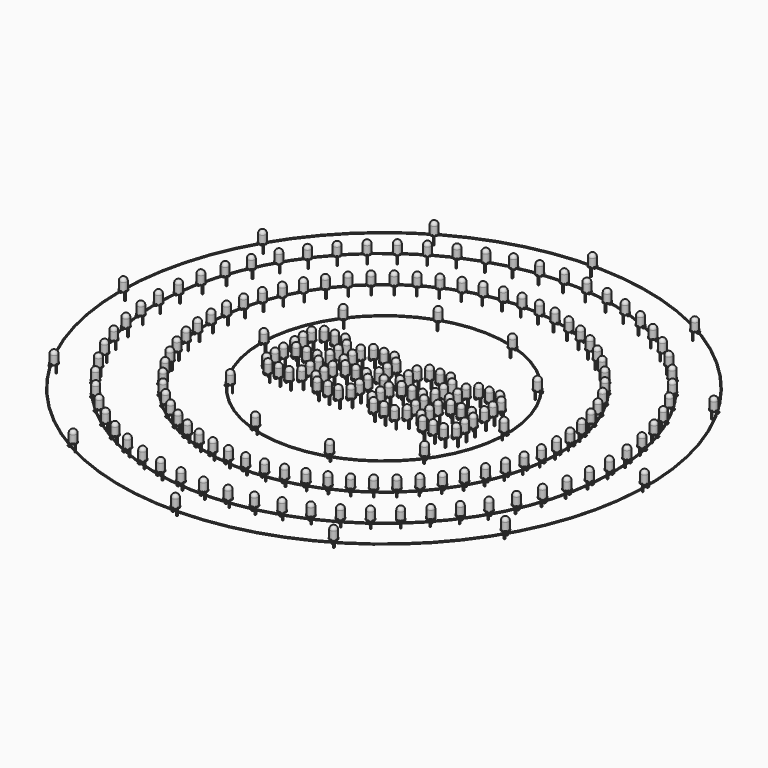
from build123d import *

# Parameters (mm, degrees)
F2_W       = 0.762
F2_H       = 0.762
F3_DEPTH   = 1.27
F4_DEPTH   = 6.35
F5_R       = 0.4064
F7_ANGLE   = 270
F3_FACE1_W = 0.762
F3_FACE1_H = 0.762
F9_ANGLE   = 180
F14_COUNT  = 10
F14_ANGLE  = 324
F15_COUNT  = 60
F15_ANGLE  = 354
F16_COUNT  = 12
F16_ANGLE  = 330


with BuildPart() as f1:
    # F0 (on Top) → F1 (revolve)
    with BuildSketch(Plane.XY):
        with BuildLine():
            Line((-2.794, 0), (0, 0))
            Line((0, 0), (0, 8.636))
            ThreePointArc((0, 8.636), (-1.7960512242, 7.8920512242), (-2.54, 6.096))
            Line((-2.54, 6.096), (-2.54, 0.508))
            Line((-2.54, 0.508), (-2.794, 0.508))
            Line((-2.794, 0.508), (-2.794, 0))
        make_face()
    revolve(axis=Axis((0, 4.318, 0), (0, -1, 0)))

    # F2 (on face) → F3 (join)
    with BuildSketch(Plane.XZ):
        with Locations((-1.27, 0)):
            Rectangle(F2_W, F2_H)
    extrude(amount=F3_DEPTH)

    # F2 (on face) → F4 (join)
    with BuildSketch(Plane.XZ):
        with Locations((1.27, 0)):
            Rectangle(F2_W, F2_H)
    extrude(amount=F4_DEPTH)


with BuildPart() as f6:
    # F5 (on Front) → F6 (revolve)
    with BuildSketch(Plane.XZ):
        with Locations((-190.5, 0)):
            Circle(F5_R)
    revolve(axis=Axis((0, 0, -20.106445998), (0, 0, -1)))


with BuildPart() as f6b:
    # F5 (on Front) → F6, piece 2 (revolve)
    with BuildSketch(Plane.XZ):
        with Locations((-165.1, 0)):
            Circle(F5_R)
    revolve(axis=Axis((0, 0, -20.106445998), (0, 0, -1)))


with BuildPart() as f6c:
    # F5 (on Front) → F6, piece 3 (revolve)
    with BuildSketch(Plane.XZ):
        with Locations((-127, 0)):
            Circle(F5_R)
    revolve(axis=Axis((0, 0, -20.106445998), (0, 0, -1)))


with BuildPart() as f6d:
    # F5 (on Front) → F6, piece 4 (revolve)
    with BuildSketch(Plane.XZ):
        with Locations((-88.9, 0)):
            Circle(F5_R)
    revolve(axis=Axis((0, 0, -20.106445998), (0, 0, -1)))


with BuildPart() as f1_1:
    # F7: moved
    add(f1.part.rotate(Axis((-1.397, 0, 0), (-1, 0, 0)), F7_ANGLE))

    # F3_face1 (on face) → F9 (revolve)
    with BuildSketch(Plane(origin=(-1.27, 0, -1.27), x_dir=(1, 0, 0), z_dir=(0, 0, -1))):
        Rectangle(F3_FACE1_W, F3_FACE1_H)
    revolve(axis=Axis((-2.0574, -0.381, -1.27), (0, 1, 0)), revolution_arc=F9_ANGLE)


with BuildPart() as f10_1:
    # F10: copy of F1
    add(f1_1.part.moved(Location((-86.868, 0, 1.27))))


with BuildPart() as f11_1:
    # F11: copy of F1
    add(f1_1.part.moved(Location((-124.968, 0, 1.27))))


with BuildPart() as f12_1:
    # F12: copy of F1
    add(f1_1.part.moved(Location((-163.068, 0, 1.27))))


with BuildPart() as f13_1:
    # F13: copy of F1
    add(f1_1.part.moved(Location((-188.468, 0, 1.27))))


with BuildPart() as f14_1:
    # F14: instance of F10_1
    add(f10_1.part.rotate(Axis((0, 0, 22.3142132163), (0, 0, -1)), 1 * F14_ANGLE / (F14_COUNT - 1)))


with BuildPart() as f14_2:
    # F14: instance of F10_1
    add(f10_1.part.rotate(Axis((0, 0, 22.3142132163), (0, 0, -1)), 2 * F14_ANGLE / (F14_COUNT - 1)))


with BuildPart() as f14_3:
    # F14: instance of F10_1
    add(f10_1.part.rotate(Axis((0, 0, 22.3142132163), (0, 0, -1)), 3 * F14_ANGLE / (F14_COUNT - 1)))


with BuildPart() as f14_4:
    # F14: instance of F10_1
    add(f10_1.part.rotate(Axis((0, 0, 22.3142132163), (0, 0, -1)), 4 * F14_ANGLE / (F14_COUNT - 1)))


with BuildPart() as f14_5:
    # F14: instance of F10_1
    add(f10_1.part.rotate(Axis((0, 0, 22.3142132163), (0, 0, -1)), 5 * F14_ANGLE / (F14_COUNT - 1)))


with BuildPart() as f14_6:
    # F14: instance of F10_1
    add(f10_1.part.rotate(Axis((0, 0, 22.3142132163), (0, 0, -1)), 6 * F14_ANGLE / (F14_COUNT - 1)))


with BuildPart() as f14_7:
    # F14: instance of F10_1
    add(f10_1.part.rotate(Axis((0, 0, 22.3142132163), (0, 0, -1)), 7 * F14_ANGLE / (F14_COUNT - 1)))


with BuildPart() as f14_8:
    # F14: instance of F10_1
    add(f10_1.part.rotate(Axis((0, 0, 22.3142132163), (0, 0, -1)), 8 * F14_ANGLE / (F14_COUNT - 1)))


with BuildPart() as f14_9:
    # F14: instance of F10_1
    add(f10_1.part.rotate(Axis((0, 0, 22.3142132163), (0, 0, -1)), 9 * F14_ANGLE / (F14_COUNT - 1)))


with BuildPart() as f15_1:
    # F15: instance of F11_1
    add(f11_1.part.rotate(Axis((0, 0, 22.3142132163), (0, 0, -1)), 1 * F15_ANGLE / (F15_COUNT - 1)))


with BuildPart() as f15_2:
    # F15: instance of F11_1
    add(f11_1.part.rotate(Axis((0, 0, 22.3142132163), (0, 0, -1)), 2 * F15_ANGLE / (F15_COUNT - 1)))


with BuildPart() as f15_3:
    # F15: instance of F11_1
    add(f11_1.part.rotate(Axis((0, 0, 22.3142132163), (0, 0, -1)), 3 * F15_ANGLE / (F15_COUNT - 1)))


with BuildPart() as f15_4:
    # F15: instance of F11_1
    add(f11_1.part.rotate(Axis((0, 0, 22.3142132163), (0, 0, -1)), 4 * F15_ANGLE / (F15_COUNT - 1)))


with BuildPart() as f15_5:
    # F15: instance of F11_1
    add(f11_1.part.rotate(Axis((0, 0, 22.3142132163), (0, 0, -1)), 5 * F15_ANGLE / (F15_COUNT - 1)))


with BuildPart() as f15_6:
    # F15: instance of F11_1
    add(f11_1.part.rotate(Axis((0, 0, 22.3142132163), (0, 0, -1)), 6 * F15_ANGLE / (F15_COUNT - 1)))


with BuildPart() as f15_7:
    # F15: instance of F11_1
    add(f11_1.part.rotate(Axis((0, 0, 22.3142132163), (0, 0, -1)), 7 * F15_ANGLE / (F15_COUNT - 1)))


with BuildPart() as f15_8:
    # F15: instance of F11_1
    add(f11_1.part.rotate(Axis((0, 0, 22.3142132163), (0, 0, -1)), 8 * F15_ANGLE / (F15_COUNT - 1)))


with BuildPart() as f15_9:
    # F15: instance of F11_1
    add(f11_1.part.rotate(Axis((0, 0, 22.3142132163), (0, 0, -1)), 9 * F15_ANGLE / (F15_COUNT - 1)))


with BuildPart() as f15_10:
    # F15: instance of F11_1
    add(f11_1.part.rotate(Axis((0, 0, 22.3142132163), (0, 0, -1)), 10 * F15_ANGLE / (F15_COUNT - 1)))


with BuildPart() as f15_11:
    # F15: instance of F11_1
    add(f11_1.part.rotate(Axis((0, 0, 22.3142132163), (0, 0, -1)), 11 * F15_ANGLE / (F15_COUNT - 1)))


with BuildPart() as f15_12:
    # F15: instance of F11_1
    add(f11_1.part.rotate(Axis((0, 0, 22.3142132163), (0, 0, -1)), 12 * F15_ANGLE / (F15_COUNT - 1)))


with BuildPart() as f15_13:
    # F15: instance of F11_1
    add(f11_1.part.rotate(Axis((0, 0, 22.3142132163), (0, 0, -1)), 13 * F15_ANGLE / (F15_COUNT - 1)))


with BuildPart() as f15_14:
    # F15: instance of F11_1
    add(f11_1.part.rotate(Axis((0, 0, 22.3142132163), (0, 0, -1)), 14 * F15_ANGLE / (F15_COUNT - 1)))


with BuildPart() as f15_15:
    # F15: instance of F11_1
    add(f11_1.part.rotate(Axis((0, 0, 22.3142132163), (0, 0, -1)), 15 * F15_ANGLE / (F15_COUNT - 1)))


with BuildPart() as f15_16:
    # F15: instance of F11_1
    add(f11_1.part.rotate(Axis((0, 0, 22.3142132163), (0, 0, -1)), 16 * F15_ANGLE / (F15_COUNT - 1)))


with BuildPart() as f15_17:
    # F15: instance of F11_1
    add(f11_1.part.rotate(Axis((0, 0, 22.3142132163), (0, 0, -1)), 17 * F15_ANGLE / (F15_COUNT - 1)))


with BuildPart() as f15_18:
    # F15: instance of F11_1
    add(f11_1.part.rotate(Axis((0, 0, 22.3142132163), (0, 0, -1)), 18 * F15_ANGLE / (F15_COUNT - 1)))


with BuildPart() as f15_19:
    # F15: instance of F11_1
    add(f11_1.part.rotate(Axis((0, 0, 22.3142132163), (0, 0, -1)), 19 * F15_ANGLE / (F15_COUNT - 1)))


with BuildPart() as f15_20:
    # F15: instance of F11_1
    add(f11_1.part.rotate(Axis((0, 0, 22.3142132163), (0, 0, -1)), 20 * F15_ANGLE / (F15_COUNT - 1)))


with BuildPart() as f15_21:
    # F15: instance of F11_1
    add(f11_1.part.rotate(Axis((0, 0, 22.3142132163), (0, 0, -1)), 21 * F15_ANGLE / (F15_COUNT - 1)))


with BuildPart() as f15_22:
    # F15: instance of F11_1
    add(f11_1.part.rotate(Axis((0, 0, 22.3142132163), (0, 0, -1)), 22 * F15_ANGLE / (F15_COUNT - 1)))


with BuildPart() as f15_23:
    # F15: instance of F11_1
    add(f11_1.part.rotate(Axis((0, 0, 22.3142132163), (0, 0, -1)), 23 * F15_ANGLE / (F15_COUNT - 1)))


with BuildPart() as f15_24:
    # F15: instance of F11_1
    add(f11_1.part.rotate(Axis((0, 0, 22.3142132163), (0, 0, -1)), 24 * F15_ANGLE / (F15_COUNT - 1)))


with BuildPart() as f15_25:
    # F15: instance of F11_1
    add(f11_1.part.rotate(Axis((0, 0, 22.3142132163), (0, 0, -1)), 25 * F15_ANGLE / (F15_COUNT - 1)))


with BuildPart() as f15_26:
    # F15: instance of F11_1
    add(f11_1.part.rotate(Axis((0, 0, 22.3142132163), (0, 0, -1)), 26 * F15_ANGLE / (F15_COUNT - 1)))


with BuildPart() as f15_27:
    # F15: instance of F11_1
    add(f11_1.part.rotate(Axis((0, 0, 22.3142132163), (0, 0, -1)), 27 * F15_ANGLE / (F15_COUNT - 1)))


with BuildPart() as f15_28:
    # F15: instance of F11_1
    add(f11_1.part.rotate(Axis((0, 0, 22.3142132163), (0, 0, -1)), 28 * F15_ANGLE / (F15_COUNT - 1)))


with BuildPart() as f15_29:
    # F15: instance of F11_1
    add(f11_1.part.rotate(Axis((0, 0, 22.3142132163), (0, 0, -1)), 29 * F15_ANGLE / (F15_COUNT - 1)))


with BuildPart() as f15_30:
    # F15: instance of F11_1
    add(f11_1.part.rotate(Axis((0, 0, 22.3142132163), (0, 0, -1)), 30 * F15_ANGLE / (F15_COUNT - 1)))


with BuildPart() as f15_31:
    # F15: instance of F11_1
    add(f11_1.part.rotate(Axis((0, 0, 22.3142132163), (0, 0, -1)), 31 * F15_ANGLE / (F15_COUNT - 1)))


with BuildPart() as f15_32:
    # F15: instance of F11_1
    add(f11_1.part.rotate(Axis((0, 0, 22.3142132163), (0, 0, -1)), 32 * F15_ANGLE / (F15_COUNT - 1)))


with BuildPart() as f15_33:
    # F15: instance of F11_1
    add(f11_1.part.rotate(Axis((0, 0, 22.3142132163), (0, 0, -1)), 33 * F15_ANGLE / (F15_COUNT - 1)))


with BuildPart() as f15_34:
    # F15: instance of F11_1
    add(f11_1.part.rotate(Axis((0, 0, 22.3142132163), (0, 0, -1)), 34 * F15_ANGLE / (F15_COUNT - 1)))


with BuildPart() as f15_35:
    # F15: instance of F11_1
    add(f11_1.part.rotate(Axis((0, 0, 22.3142132163), (0, 0, -1)), 35 * F15_ANGLE / (F15_COUNT - 1)))


with BuildPart() as f15_36:
    # F15: instance of F11_1
    add(f11_1.part.rotate(Axis((0, 0, 22.3142132163), (0, 0, -1)), 36 * F15_ANGLE / (F15_COUNT - 1)))


with BuildPart() as f15_37:
    # F15: instance of F11_1
    add(f11_1.part.rotate(Axis((0, 0, 22.3142132163), (0, 0, -1)), 37 * F15_ANGLE / (F15_COUNT - 1)))


with BuildPart() as f15_38:
    # F15: instance of F11_1
    add(f11_1.part.rotate(Axis((0, 0, 22.3142132163), (0, 0, -1)), 38 * F15_ANGLE / (F15_COUNT - 1)))


with BuildPart() as f15_39:
    # F15: instance of F11_1
    add(f11_1.part.rotate(Axis((0, 0, 22.3142132163), (0, 0, -1)), 39 * F15_ANGLE / (F15_COUNT - 1)))


with BuildPart() as f15_40:
    # F15: instance of F11_1
    add(f11_1.part.rotate(Axis((0, 0, 22.3142132163), (0, 0, -1)), 40 * F15_ANGLE / (F15_COUNT - 1)))


with BuildPart() as f15_41:
    # F15: instance of F11_1
    add(f11_1.part.rotate(Axis((0, 0, 22.3142132163), (0, 0, -1)), 41 * F15_ANGLE / (F15_COUNT - 1)))


with BuildPart() as f15_42:
    # F15: instance of F11_1
    add(f11_1.part.rotate(Axis((0, 0, 22.3142132163), (0, 0, -1)), 42 * F15_ANGLE / (F15_COUNT - 1)))


with BuildPart() as f15_43:
    # F15: instance of F11_1
    add(f11_1.part.rotate(Axis((0, 0, 22.3142132163), (0, 0, -1)), 43 * F15_ANGLE / (F15_COUNT - 1)))


with BuildPart() as f15_44:
    # F15: instance of F11_1
    add(f11_1.part.rotate(Axis((0, 0, 22.3142132163), (0, 0, -1)), 44 * F15_ANGLE / (F15_COUNT - 1)))


with BuildPart() as f15_45:
    # F15: instance of F11_1
    add(f11_1.part.rotate(Axis((0, 0, 22.3142132163), (0, 0, -1)), 45 * F15_ANGLE / (F15_COUNT - 1)))


with BuildPart() as f15_46:
    # F15: instance of F11_1
    add(f11_1.part.rotate(Axis((0, 0, 22.3142132163), (0, 0, -1)), 46 * F15_ANGLE / (F15_COUNT - 1)))


with BuildPart() as f15_47:
    # F15: instance of F11_1
    add(f11_1.part.rotate(Axis((0, 0, 22.3142132163), (0, 0, -1)), 47 * F15_ANGLE / (F15_COUNT - 1)))


with BuildPart() as f15_48:
    # F15: instance of F11_1
    add(f11_1.part.rotate(Axis((0, 0, 22.3142132163), (0, 0, -1)), 48 * F15_ANGLE / (F15_COUNT - 1)))


with BuildPart() as f15_49:
    # F15: instance of F11_1
    add(f11_1.part.rotate(Axis((0, 0, 22.3142132163), (0, 0, -1)), 49 * F15_ANGLE / (F15_COUNT - 1)))


with BuildPart() as f15_50:
    # F15: instance of F11_1
    add(f11_1.part.rotate(Axis((0, 0, 22.3142132163), (0, 0, -1)), 50 * F15_ANGLE / (F15_COUNT - 1)))


with BuildPart() as f15_51:
    # F15: instance of F11_1
    add(f11_1.part.rotate(Axis((0, 0, 22.3142132163), (0, 0, -1)), 51 * F15_ANGLE / (F15_COUNT - 1)))


with BuildPart() as f15_52:
    # F15: instance of F11_1
    add(f11_1.part.rotate(Axis((0, 0, 22.3142132163), (0, 0, -1)), 52 * F15_ANGLE / (F15_COUNT - 1)))


with BuildPart() as f15_53:
    # F15: instance of F11_1
    add(f11_1.part.rotate(Axis((0, 0, 22.3142132163), (0, 0, -1)), 53 * F15_ANGLE / (F15_COUNT - 1)))


with BuildPart() as f15_54:
    # F15: instance of F11_1
    add(f11_1.part.rotate(Axis((0, 0, 22.3142132163), (0, 0, -1)), 54 * F15_ANGLE / (F15_COUNT - 1)))


with BuildPart() as f15_55:
    # F15: instance of F11_1
    add(f11_1.part.rotate(Axis((0, 0, 22.3142132163), (0, 0, -1)), 55 * F15_ANGLE / (F15_COUNT - 1)))


with BuildPart() as f15_56:
    # F15: instance of F11_1
    add(f11_1.part.rotate(Axis((0, 0, 22.3142132163), (0, 0, -1)), 56 * F15_ANGLE / (F15_COUNT - 1)))


with BuildPart() as f15_57:
    # F15: instance of F11_1
    add(f11_1.part.rotate(Axis((0, 0, 22.3142132163), (0, 0, -1)), 57 * F15_ANGLE / (F15_COUNT - 1)))


with BuildPart() as f15_58:
    # F15: instance of F11_1
    add(f11_1.part.rotate(Axis((0, 0, 22.3142132163), (0, 0, -1)), 58 * F15_ANGLE / (F15_COUNT - 1)))


with BuildPart() as f15_59:
    # F15: instance of F11_1
    add(f11_1.part.rotate(Axis((0, 0, 22.3142132163), (0, 0, -1)), 59 * F15_ANGLE / (F15_COUNT - 1)))


with BuildPart() as f15_60:
    # F15: instance of F12_1
    add(f12_1.part.rotate(Axis((0, 0, 22.3142132163), (0, 0, -1)), 1 * F15_ANGLE / (F15_COUNT - 1)))


with BuildPart() as f15_61:
    # F15: instance of F12_1
    add(f12_1.part.rotate(Axis((0, 0, 22.3142132163), (0, 0, -1)), 2 * F15_ANGLE / (F15_COUNT - 1)))


with BuildPart() as f15_62:
    # F15: instance of F12_1
    add(f12_1.part.rotate(Axis((0, 0, 22.3142132163), (0, 0, -1)), 3 * F15_ANGLE / (F15_COUNT - 1)))


with BuildPart() as f15_63:
    # F15: instance of F12_1
    add(f12_1.part.rotate(Axis((0, 0, 22.3142132163), (0, 0, -1)), 4 * F15_ANGLE / (F15_COUNT - 1)))


with BuildPart() as f15_64:
    # F15: instance of F12_1
    add(f12_1.part.rotate(Axis((0, 0, 22.3142132163), (0, 0, -1)), 5 * F15_ANGLE / (F15_COUNT - 1)))


with BuildPart() as f15_65:
    # F15: instance of F12_1
    add(f12_1.part.rotate(Axis((0, 0, 22.3142132163), (0, 0, -1)), 6 * F15_ANGLE / (F15_COUNT - 1)))


with BuildPart() as f15_66:
    # F15: instance of F12_1
    add(f12_1.part.rotate(Axis((0, 0, 22.3142132163), (0, 0, -1)), 7 * F15_ANGLE / (F15_COUNT - 1)))


with BuildPart() as f15_67:
    # F15: instance of F12_1
    add(f12_1.part.rotate(Axis((0, 0, 22.3142132163), (0, 0, -1)), 8 * F15_ANGLE / (F15_COUNT - 1)))


with BuildPart() as f15_68:
    # F15: instance of F12_1
    add(f12_1.part.rotate(Axis((0, 0, 22.3142132163), (0, 0, -1)), 9 * F15_ANGLE / (F15_COUNT - 1)))


with BuildPart() as f15_69:
    # F15: instance of F12_1
    add(f12_1.part.rotate(Axis((0, 0, 22.3142132163), (0, 0, -1)), 10 * F15_ANGLE / (F15_COUNT - 1)))


with BuildPart() as f15_70:
    # F15: instance of F12_1
    add(f12_1.part.rotate(Axis((0, 0, 22.3142132163), (0, 0, -1)), 11 * F15_ANGLE / (F15_COUNT - 1)))


with BuildPart() as f15_71:
    # F15: instance of F12_1
    add(f12_1.part.rotate(Axis((0, 0, 22.3142132163), (0, 0, -1)), 12 * F15_ANGLE / (F15_COUNT - 1)))


with BuildPart() as f15_72:
    # F15: instance of F12_1
    add(f12_1.part.rotate(Axis((0, 0, 22.3142132163), (0, 0, -1)), 13 * F15_ANGLE / (F15_COUNT - 1)))


with BuildPart() as f15_73:
    # F15: instance of F12_1
    add(f12_1.part.rotate(Axis((0, 0, 22.3142132163), (0, 0, -1)), 14 * F15_ANGLE / (F15_COUNT - 1)))


with BuildPart() as f15_74:
    # F15: instance of F12_1
    add(f12_1.part.rotate(Axis((0, 0, 22.3142132163), (0, 0, -1)), 15 * F15_ANGLE / (F15_COUNT - 1)))


with BuildPart() as f15_75:
    # F15: instance of F12_1
    add(f12_1.part.rotate(Axis((0, 0, 22.3142132163), (0, 0, -1)), 16 * F15_ANGLE / (F15_COUNT - 1)))


with BuildPart() as f15_76:
    # F15: instance of F12_1
    add(f12_1.part.rotate(Axis((0, 0, 22.3142132163), (0, 0, -1)), 17 * F15_ANGLE / (F15_COUNT - 1)))


with BuildPart() as f15_77:
    # F15: instance of F12_1
    add(f12_1.part.rotate(Axis((0, 0, 22.3142132163), (0, 0, -1)), 18 * F15_ANGLE / (F15_COUNT - 1)))


with BuildPart() as f15_78:
    # F15: instance of F12_1
    add(f12_1.part.rotate(Axis((0, 0, 22.3142132163), (0, 0, -1)), 19 * F15_ANGLE / (F15_COUNT - 1)))


with BuildPart() as f15_79:
    # F15: instance of F12_1
    add(f12_1.part.rotate(Axis((0, 0, 22.3142132163), (0, 0, -1)), 20 * F15_ANGLE / (F15_COUNT - 1)))


with BuildPart() as f15_80:
    # F15: instance of F12_1
    add(f12_1.part.rotate(Axis((0, 0, 22.3142132163), (0, 0, -1)), 21 * F15_ANGLE / (F15_COUNT - 1)))


with BuildPart() as f15_81:
    # F15: instance of F12_1
    add(f12_1.part.rotate(Axis((0, 0, 22.3142132163), (0, 0, -1)), 22 * F15_ANGLE / (F15_COUNT - 1)))


with BuildPart() as f15_82:
    # F15: instance of F12_1
    add(f12_1.part.rotate(Axis((0, 0, 22.3142132163), (0, 0, -1)), 23 * F15_ANGLE / (F15_COUNT - 1)))


with BuildPart() as f15_83:
    # F15: instance of F12_1
    add(f12_1.part.rotate(Axis((0, 0, 22.3142132163), (0, 0, -1)), 24 * F15_ANGLE / (F15_COUNT - 1)))


with BuildPart() as f15_84:
    # F15: instance of F12_1
    add(f12_1.part.rotate(Axis((0, 0, 22.3142132163), (0, 0, -1)), 25 * F15_ANGLE / (F15_COUNT - 1)))


with BuildPart() as f15_85:
    # F15: instance of F12_1
    add(f12_1.part.rotate(Axis((0, 0, 22.3142132163), (0, 0, -1)), 26 * F15_ANGLE / (F15_COUNT - 1)))


with BuildPart() as f15_86:
    # F15: instance of F12_1
    add(f12_1.part.rotate(Axis((0, 0, 22.3142132163), (0, 0, -1)), 27 * F15_ANGLE / (F15_COUNT - 1)))


with BuildPart() as f15_87:
    # F15: instance of F12_1
    add(f12_1.part.rotate(Axis((0, 0, 22.3142132163), (0, 0, -1)), 28 * F15_ANGLE / (F15_COUNT - 1)))


with BuildPart() as f15_88:
    # F15: instance of F12_1
    add(f12_1.part.rotate(Axis((0, 0, 22.3142132163), (0, 0, -1)), 29 * F15_ANGLE / (F15_COUNT - 1)))


with BuildPart() as f15_89:
    # F15: instance of F12_1
    add(f12_1.part.rotate(Axis((0, 0, 22.3142132163), (0, 0, -1)), 30 * F15_ANGLE / (F15_COUNT - 1)))


with BuildPart() as f15_90:
    # F15: instance of F12_1
    add(f12_1.part.rotate(Axis((0, 0, 22.3142132163), (0, 0, -1)), 31 * F15_ANGLE / (F15_COUNT - 1)))


with BuildPart() as f15_91:
    # F15: instance of F12_1
    add(f12_1.part.rotate(Axis((0, 0, 22.3142132163), (0, 0, -1)), 32 * F15_ANGLE / (F15_COUNT - 1)))


with BuildPart() as f15_92:
    # F15: instance of F12_1
    add(f12_1.part.rotate(Axis((0, 0, 22.3142132163), (0, 0, -1)), 33 * F15_ANGLE / (F15_COUNT - 1)))


with BuildPart() as f15_93:
    # F15: instance of F12_1
    add(f12_1.part.rotate(Axis((0, 0, 22.3142132163), (0, 0, -1)), 34 * F15_ANGLE / (F15_COUNT - 1)))


with BuildPart() as f15_94:
    # F15: instance of F12_1
    add(f12_1.part.rotate(Axis((0, 0, 22.3142132163), (0, 0, -1)), 35 * F15_ANGLE / (F15_COUNT - 1)))


with BuildPart() as f15_95:
    # F15: instance of F12_1
    add(f12_1.part.rotate(Axis((0, 0, 22.3142132163), (0, 0, -1)), 36 * F15_ANGLE / (F15_COUNT - 1)))


with BuildPart() as f15_96:
    # F15: instance of F12_1
    add(f12_1.part.rotate(Axis((0, 0, 22.3142132163), (0, 0, -1)), 37 * F15_ANGLE / (F15_COUNT - 1)))


with BuildPart() as f15_97:
    # F15: instance of F12_1
    add(f12_1.part.rotate(Axis((0, 0, 22.3142132163), (0, 0, -1)), 38 * F15_ANGLE / (F15_COUNT - 1)))


with BuildPart() as f15_98:
    # F15: instance of F12_1
    add(f12_1.part.rotate(Axis((0, 0, 22.3142132163), (0, 0, -1)), 39 * F15_ANGLE / (F15_COUNT - 1)))


with BuildPart() as f15_99:
    # F15: instance of F12_1
    add(f12_1.part.rotate(Axis((0, 0, 22.3142132163), (0, 0, -1)), 40 * F15_ANGLE / (F15_COUNT - 1)))


with BuildPart() as f15_100:
    # F15: instance of F12_1
    add(f12_1.part.rotate(Axis((0, 0, 22.3142132163), (0, 0, -1)), 41 * F15_ANGLE / (F15_COUNT - 1)))


with BuildPart() as f15_101:
    # F15: instance of F12_1
    add(f12_1.part.rotate(Axis((0, 0, 22.3142132163), (0, 0, -1)), 42 * F15_ANGLE / (F15_COUNT - 1)))


with BuildPart() as f15_102:
    # F15: instance of F12_1
    add(f12_1.part.rotate(Axis((0, 0, 22.3142132163), (0, 0, -1)), 43 * F15_ANGLE / (F15_COUNT - 1)))


with BuildPart() as f15_103:
    # F15: instance of F12_1
    add(f12_1.part.rotate(Axis((0, 0, 22.3142132163), (0, 0, -1)), 44 * F15_ANGLE / (F15_COUNT - 1)))


with BuildPart() as f15_104:
    # F15: instance of F12_1
    add(f12_1.part.rotate(Axis((0, 0, 22.3142132163), (0, 0, -1)), 45 * F15_ANGLE / (F15_COUNT - 1)))


with BuildPart() as f15_105:
    # F15: instance of F12_1
    add(f12_1.part.rotate(Axis((0, 0, 22.3142132163), (0, 0, -1)), 46 * F15_ANGLE / (F15_COUNT - 1)))


with BuildPart() as f15_106:
    # F15: instance of F12_1
    add(f12_1.part.rotate(Axis((0, 0, 22.3142132163), (0, 0, -1)), 47 * F15_ANGLE / (F15_COUNT - 1)))


with BuildPart() as f15_107:
    # F15: instance of F12_1
    add(f12_1.part.rotate(Axis((0, 0, 22.3142132163), (0, 0, -1)), 48 * F15_ANGLE / (F15_COUNT - 1)))


with BuildPart() as f15_108:
    # F15: instance of F12_1
    add(f12_1.part.rotate(Axis((0, 0, 22.3142132163), (0, 0, -1)), 49 * F15_ANGLE / (F15_COUNT - 1)))


with BuildPart() as f15_109:
    # F15: instance of F12_1
    add(f12_1.part.rotate(Axis((0, 0, 22.3142132163), (0, 0, -1)), 50 * F15_ANGLE / (F15_COUNT - 1)))


with BuildPart() as f15_110:
    # F15: instance of F12_1
    add(f12_1.part.rotate(Axis((0, 0, 22.3142132163), (0, 0, -1)), 51 * F15_ANGLE / (F15_COUNT - 1)))


with BuildPart() as f15_111:
    # F15: instance of F12_1
    add(f12_1.part.rotate(Axis((0, 0, 22.3142132163), (0, 0, -1)), 52 * F15_ANGLE / (F15_COUNT - 1)))


with BuildPart() as f15_112:
    # F15: instance of F12_1
    add(f12_1.part.rotate(Axis((0, 0, 22.3142132163), (0, 0, -1)), 53 * F15_ANGLE / (F15_COUNT - 1)))


with BuildPart() as f15_113:
    # F15: instance of F12_1
    add(f12_1.part.rotate(Axis((0, 0, 22.3142132163), (0, 0, -1)), 54 * F15_ANGLE / (F15_COUNT - 1)))


with BuildPart() as f15_114:
    # F15: instance of F12_1
    add(f12_1.part.rotate(Axis((0, 0, 22.3142132163), (0, 0, -1)), 55 * F15_ANGLE / (F15_COUNT - 1)))


with BuildPart() as f15_115:
    # F15: instance of F12_1
    add(f12_1.part.rotate(Axis((0, 0, 22.3142132163), (0, 0, -1)), 56 * F15_ANGLE / (F15_COUNT - 1)))


with BuildPart() as f15_116:
    # F15: instance of F12_1
    add(f12_1.part.rotate(Axis((0, 0, 22.3142132163), (0, 0, -1)), 57 * F15_ANGLE / (F15_COUNT - 1)))


with BuildPart() as f15_117:
    # F15: instance of F12_1
    add(f12_1.part.rotate(Axis((0, 0, 22.3142132163), (0, 0, -1)), 58 * F15_ANGLE / (F15_COUNT - 1)))


with BuildPart() as f15_118:
    # F15: instance of F12_1
    add(f12_1.part.rotate(Axis((0, 0, 22.3142132163), (0, 0, -1)), 59 * F15_ANGLE / (F15_COUNT - 1)))


with BuildPart() as f16_1:
    # F16: instance of F13_1
    add(f13_1.part.rotate(Axis((0, 0, 22.3142132163), (0, 0, -1)), 1 * F16_ANGLE / (F16_COUNT - 1)))


with BuildPart() as f16_2:
    # F16: instance of F13_1
    add(f13_1.part.rotate(Axis((0, 0, 22.3142132163), (0, 0, -1)), 2 * F16_ANGLE / (F16_COUNT - 1)))


with BuildPart() as f16_3:
    # F16: instance of F13_1
    add(f13_1.part.rotate(Axis((0, 0, 22.3142132163), (0, 0, -1)), 3 * F16_ANGLE / (F16_COUNT - 1)))


with BuildPart() as f16_4:
    # F16: instance of F13_1
    add(f13_1.part.rotate(Axis((0, 0, 22.3142132163), (0, 0, -1)), 4 * F16_ANGLE / (F16_COUNT - 1)))


with BuildPart() as f16_5:
    # F16: instance of F13_1
    add(f13_1.part.rotate(Axis((0, 0, 22.3142132163), (0, 0, -1)), 5 * F16_ANGLE / (F16_COUNT - 1)))


with BuildPart() as f16_6:
    # F16: instance of F13_1
    add(f13_1.part.rotate(Axis((0, 0, 22.3142132163), (0, 0, -1)), 6 * F16_ANGLE / (F16_COUNT - 1)))


with BuildPart() as f16_7:
    # F16: instance of F13_1
    add(f13_1.part.rotate(Axis((0, 0, 22.3142132163), (0, 0, -1)), 7 * F16_ANGLE / (F16_COUNT - 1)))


with BuildPart() as f16_8:
    # F16: instance of F13_1
    add(f13_1.part.rotate(Axis((0, 0, 22.3142132163), (0, 0, -1)), 8 * F16_ANGLE / (F16_COUNT - 1)))


with BuildPart() as f16_9:
    # F16: instance of F13_1
    add(f13_1.part.rotate(Axis((0, 0, 22.3142132163), (0, 0, -1)), 9 * F16_ANGLE / (F16_COUNT - 1)))


with BuildPart() as f16_10:
    # F16: instance of F13_1
    add(f13_1.part.rotate(Axis((0, 0, 22.3142132163), (0, 0, -1)), 10 * F16_ANGLE / (F16_COUNT - 1)))


with BuildPart() as f16_11:
    # F16: instance of F13_1
    add(f13_1.part.rotate(Axis((0, 0, 22.3142132163), (0, 0, -1)), 11 * F16_ANGLE / (F16_COUNT - 1)))


with BuildPart() as f17_1:
    # F17: copy of F1
    add(f1_1.part.moved(Location((-63.5, 0, 0))))


with BuildPart() as f18_1:
    # F18: copy of F17_1
    add(f17_1.part.moved(Location((7.62, 0, 0))))


with BuildPart() as f19_1:
    # F19: copy of F18_1
    add(f18_1.part.moved(Location((7.62, 0, 0))))


with BuildPart() as f20_1:
    # F20: copy of F17_1
    add(f17_1.part.moved(Location((0, -25.4, 0))))


with BuildPart() as f20_2:
    # F20: copy of F19_1
    add(f19_1.part.moved(Location((0, -25.4, 0))))


with BuildPart() as f20_3:
    # F20: copy of F18_1
    add(f18_1.part.moved(Location((0, -25.4, 0))))


with BuildPart() as f21_1:
    # F21: copy of F17_1
    add(f17_1.part.moved(Location((0, 25.4, 0))))


with BuildPart() as f21_2:
    # F21: copy of F18_1
    add(f18_1.part.moved(Location((0, 25.4, 0))))


with BuildPart() as f21_3:
    # F21: copy of F19_1
    add(f19_1.part.moved(Location((0, 25.4, 0))))


with BuildPart() as f22_1:
    # F22: copy of F1
    add(f1_1.part.moved(Location((-68.58, 5.08, 0))))


with BuildPart() as f23_1:
    # F23: copy of F22_1
    add(f22_1.part.moved(Location((0, 7.62, 0))))


with BuildPart() as f24_1:
    # F24: copy of F23_1
    add(f23_1.part.moved(Location((0, 7.62, 0))))


with BuildPart() as f25_1:
    # F25: copy of F24_1
    add(f24_1.part.moved(Location((25.4, 0, 0))))


with BuildPart() as f25_2:
    # F25: copy of F23_1
    add(f23_1.part.moved(Location((25.4, 0, 0))))


with BuildPart() as f25_3:
    # F25: copy of F22_1
    add(f22_1.part.moved(Location((25.4, 0, 0))))


with BuildPart() as f26_1:
    # F26: copy of F25_1
    add(f25_1.part.moved(Location((0, -25.4, 0))))


with BuildPart() as f26_2:
    # F26: copy of F25_2
    add(f25_2.part.moved(Location((0, -25.4, 0))))


with BuildPart() as f26_3:
    # F26: copy of F25_3
    add(f25_3.part.moved(Location((0, -25.4, 0))))


with BuildPart() as f26_4:
    # F26: copy of F22_1
    add(f22_1.part.moved(Location((0, -25.4, 0))))


with BuildPart() as f26_5:
    # F26: copy of F23_1
    add(f23_1.part.moved(Location((0, -25.4, 0))))


with BuildPart() as f26_6:
    # F26: copy of F24_1
    add(f24_1.part.moved(Location((0, -25.4, 0))))


with BuildPart() as f27_1:
    # F27: copy of F21_1
    add(f21_1.part.moved(Location((35.56, 0, 0))))


with BuildPart() as f27_2:
    # F27: copy of F25_1
    add(f25_1.part.moved(Location((35.56, 0, 0))))


with BuildPart() as f27_3:
    # F27: copy of F25_2
    add(f25_2.part.moved(Location((35.56, 0, 0))))


with BuildPart() as f27_4:
    # F27: copy of F25_3
    add(f25_3.part.moved(Location((35.56, 0, 0))))


with BuildPart() as f27_5:
    # F27: copy of F19_1
    add(f19_1.part.moved(Location((35.56, 0, 0))))


with BuildPart() as f27_6:
    # F27: copy of F18_1
    add(f18_1.part.moved(Location((35.56, 0, 0))))


with BuildPart() as f27_7:
    # F27: copy of F17_1
    add(f17_1.part.moved(Location((35.56, 0, 0))))


with BuildPart() as f27_8:
    # F27: copy of F22_1
    add(f22_1.part.moved(Location((35.56, 0, 0))))


with BuildPart() as f27_9:
    # F27: copy of F23_1
    add(f23_1.part.moved(Location((35.56, 0, 0))))


with BuildPart() as f27_10:
    # F27: copy of F24_1
    add(f24_1.part.moved(Location((35.56, 0, 0))))


with BuildPart() as f27_11:
    # F27: copy of F21_3
    add(f21_3.part.moved(Location((35.56, 0, 0))))


with BuildPart() as f27_12:
    # F27: copy of F20_2
    add(f20_2.part.moved(Location((35.56, 0, 0))))


with BuildPart() as f27_13:
    # F27: copy of F20_3
    add(f20_3.part.moved(Location((35.56, 0, 0))))


with BuildPart() as f27_14:
    # F27: copy of F20_1
    add(f20_1.part.moved(Location((35.56, 0, 0))))


with BuildPart() as f27_15:
    # F27: copy of F21_2
    add(f21_2.part.moved(Location((35.56, 0, 0))))


with BuildPart() as f27_16:
    # F27: copy of F26_1
    add(f26_1.part.moved(Location((35.56, 0, 0))))


with BuildPart() as f27_17:
    # F27: copy of F26_2
    add(f26_2.part.moved(Location((35.56, 0, 0))))


with BuildPart() as f27_18:
    # F27: copy of F26_3
    add(f26_3.part.moved(Location((35.56, 0, 0))))


with BuildPart() as f27_19:
    # F27: copy of F26_4
    add(f26_4.part.moved(Location((35.56, 0, 0))))


with BuildPart() as f27_20:
    # F27: copy of F26_6
    add(f26_6.part.moved(Location((35.56, 0, 0))))


with BuildPart() as f27_21:
    # F27: copy of F26_5
    add(f26_5.part.moved(Location((35.56, 0, 0))))


with BuildPart() as f28_1:
    # F28: copy of F18_1
    add(f18_1.part.moved(Location((76.2, 0, 0))))


with BuildPart() as f28_2:
    # F28: copy of F17_1
    add(f17_1.part.moved(Location((76.2, 0, 0))))


with BuildPart() as f28_3:
    # F28: copy of F19_1
    add(f19_1.part.moved(Location((76.2, 0, 0))))


with BuildPart() as f28_4:
    # F28: copy of F20_3
    add(f20_3.part.moved(Location((76.2, 0, 0))))


with BuildPart() as f28_5:
    # F28: copy of F20_2
    add(f20_2.part.moved(Location((76.2, 0, 0))))


with BuildPart() as f28_6:
    # F28: copy of F20_1
    add(f20_1.part.moved(Location((76.2, 0, 0))))


with BuildPart() as f28_7:
    # F28: copy of F21_3
    add(f21_3.part.moved(Location((76.2, 0, 0))))


with BuildPart() as f28_8:
    # F28: copy of F21_2
    add(f21_2.part.moved(Location((76.2, 0, 0))))


with BuildPart() as f28_9:
    # F28: copy of F21_1
    add(f21_1.part.moved(Location((76.2, 0, 0))))


with BuildPart() as f28_10:
    # F28: copy of F22_1
    add(f22_1.part.moved(Location((76.2, 0, 0))))


with BuildPart() as f28_11:
    # F28: copy of F23_1
    add(f23_1.part.moved(Location((76.2, 0, 0))))


with BuildPart() as f28_12:
    # F28: copy of F24_1
    add(f24_1.part.moved(Location((76.2, 0, 0))))


with BuildPart() as f28_13:
    # F28: copy of F25_1
    add(f25_1.part.moved(Location((76.2, 0, 0))))


with BuildPart() as f28_14:
    # F28: copy of F25_2
    add(f25_2.part.moved(Location((76.2, 0, 0))))


with BuildPart() as f28_15:
    # F28: copy of F25_3
    add(f25_3.part.moved(Location((76.2, 0, 0))))


with BuildPart() as f28_16:
    # F28: copy of F26_1
    add(f26_1.part.moved(Location((76.2, 0, 0))))


with BuildPart() as f28_17:
    # F28: copy of F26_2
    add(f26_2.part.moved(Location((76.2, 0, 0))))


with BuildPart() as f28_18:
    # F28: copy of F26_3
    add(f26_3.part.moved(Location((76.2, 0, 0))))


with BuildPart() as f28_19:
    # F28: copy of F26_6
    add(f26_6.part.moved(Location((76.2, 0, 0))))


with BuildPart() as f28_20:
    # F28: copy of F26_5
    add(f26_5.part.moved(Location((76.2, 0, 0))))


with BuildPart() as f28_21:
    # F28: copy of F26_4
    add(f26_4.part.moved(Location((76.2, 0, 0))))


with BuildPart() as f28_22:
    # F28: copy of F27_13
    add(f27_13.part.moved(Location((76.2, 0, 0))))


with BuildPart() as f28_23:
    # F28: copy of F27_14
    add(f27_14.part.moved(Location((76.2, 0, 0))))


with BuildPart() as f28_24:
    # F28: copy of F27_15
    add(f27_15.part.moved(Location((76.2, 0, 0))))


with BuildPart() as f28_25:
    # F28: copy of F27_1
    add(f27_1.part.moved(Location((76.2, 0, 0))))


with BuildPart() as f28_26:
    # F28: copy of F27_12
    add(f27_12.part.moved(Location((76.2, 0, 0))))


with BuildPart() as f28_27:
    # F28: copy of F27_11
    add(f27_11.part.moved(Location((76.2, 0, 0))))


with BuildPart() as f28_28:
    # F28: copy of F27_17
    add(f27_17.part.moved(Location((76.2, 0, 0))))


with BuildPart() as f28_29:
    # F28: copy of F27_16
    add(f27_16.part.moved(Location((76.2, 0, 0))))


with BuildPart() as f28_30:
    # F28: copy of F27_5
    add(f27_5.part.moved(Location((76.2, 0, 0))))


with BuildPart() as f28_31:
    # F28: copy of F27_10
    add(f27_10.part.moved(Location((76.2, 0, 0))))


with BuildPart() as f28_32:
    # F28: copy of F27_9
    add(f27_9.part.moved(Location((76.2, 0, 0))))


with BuildPart() as f28_33:
    # F28: copy of F27_18
    add(f27_18.part.moved(Location((76.2, 0, 0))))


with BuildPart() as f28_34:
    # F28: copy of F27_8
    add(f27_8.part.moved(Location((76.2, 0, 0))))


with BuildPart() as f28_35:
    # F28: copy of F27_4
    add(f27_4.part.moved(Location((76.2, 0, 0))))


with BuildPart() as f28_36:
    # F28: copy of F27_6
    add(f27_6.part.moved(Location((76.2, 0, 0))))


with BuildPart() as f28_37:
    # F28: copy of F27_2
    add(f27_2.part.moved(Location((76.2, 0, 0))))


with BuildPart() as f28_38:
    # F28: copy of F27_3
    add(f27_3.part.moved(Location((76.2, 0, 0))))


with BuildPart() as f28_39:
    # F28: copy of F27_19
    add(f27_19.part.moved(Location((76.2, 0, 0))))


with BuildPart() as f28_40:
    # F28: copy of F27_7
    add(f27_7.part.moved(Location((76.2, 0, 0))))


with BuildPart() as f28_41:
    # F28: copy of F27_21
    add(f27_21.part.moved(Location((76.2, 0, 0))))


with BuildPart() as f28_42:
    # F28: copy of F27_20
    add(f27_20.part.moved(Location((76.2, 0, 0))))


solid = Compound([f6.part, f6b.part, f6c.part, f6d.part, f1_1.part, f10_1.part, f11_1.part, f12_1.part, f13_1.part, f14_1.part, f14_2.part, f14_3.part, f14_4.part, f14_5.part, f14_6.part, f14_7.part, f14_8.part, f14_9.part, f15_1.part, f15_2.part, f15_3.part, f15_4.part, f15_5.part, f15_6.part, f15_7.part, f15_8.part, f15_9.part, f15_10.part, f15_11.part, f15_12.part, f15_13.part, f15_14.part, f15_15.part, f15_16.part, f15_17.part, f15_18.part, f15_19.part, f15_20.part, f15_21.part, f15_22.part, f15_23.part, f15_24.part, f15_25.part, f15_26.part, f15_27.part, f15_28.part, f15_29.part, f15_30.part, f15_31.part, f15_32.part, f15_33.part, f15_34.part, f15_35.part, f15_36.part, f15_37.part, f15_38.part, f15_39.part, f15_40.part, f15_41.part, f15_42.part, f15_43.part, f15_44.part, f15_45.part, f15_46.part, f15_47.part, f15_48.part, f15_49.part, f15_50.part, f15_51.part, f15_52.part, f15_53.part, f15_54.part, f15_55.part, f15_56.part, f15_57.part, f15_58.part, f15_59.part, f15_60.part, f15_61.part, f15_62.part, f15_63.part, f15_64.part, f15_65.part, f15_66.part, f15_67.part, f15_68.part, f15_69.part, f15_70.part, f15_71.part, f15_72.part, f15_73.part, f15_74.part, f15_75.part, f15_76.part, f15_77.part, f15_78.part, f15_79.part, f15_80.part, f15_81.part, f15_82.part, f15_83.part, f15_84.part, f15_85.part, f15_86.part, f15_87.part, f15_88.part, f15_89.part, f15_90.part, f15_91.part, f15_92.part, f15_93.part, f15_94.part, f15_95.part, f15_96.part, f15_97.part, f15_98.part, f15_99.part, f15_100.part, f15_101.part, f15_102.part, f15_103.part, f15_104.part, f15_105.part, f15_106.part, f15_107.part, f15_108.part, f15_109.part, f15_110.part, f15_111.part, f15_112.part, f15_113.part, f15_114.part, f15_115.part, f15_116.part, f15_117.part, f15_118.part, f16_1.part, f16_2.part, f16_3.part, f16_4.part, f16_5.part, f16_6.part, f16_7.part, f16_8.part, f16_9.part, f16_10.part, f16_11.part, f17_1.part, f18_1.part, f19_1.part, f20_1.part, f20_2.part, f20_3.part, f21_1.part, f21_2.part, f21_3.part, f22_1.part, f23_1.part, f24_1.part, f25_1.part, f25_2.part, f25_3.part, f26_1.part, f26_2.part, f26_3.part, f26_4.part, f26_5.part, f26_6.part, f27_1.part, f27_2.part, f27_3.part, f27_4.part, f27_5.part, f27_6.part, f27_7.part, f27_8.part, f27_9.part, f27_10.part, f27_11.part, f27_12.part, f27_13.part, f27_14.part, f27_15.part, f27_16.part, f27_17.part, f27_18.part, f27_19.part, f27_20.part, f27_21.part, f28_1.part, f28_2.part, f28_3.part, f28_4.part, f28_5.part, f28_6.part, f28_7.part, f28_8.part, f28_9.part, f28_10.part, f28_11.part, f28_12.part, f28_13.part, f28_14.part, f28_15.part, f28_16.part, f28_17.part, f28_18.part, f28_19.part, f28_20.part, f28_21.part, f28_22.part, f28_23.part, f28_24.part, f28_25.part, f28_26.part, f28_27.part, f28_28.part, f28_29.part, f28_30.part, f28_31.part, f28_32.part, f28_33.part, f28_34.part, f28_35.part, f28_36.part, f28_37.part, f28_38.part, f28_39.part, f28_40.part, f28_41.part, f28_42.part])
